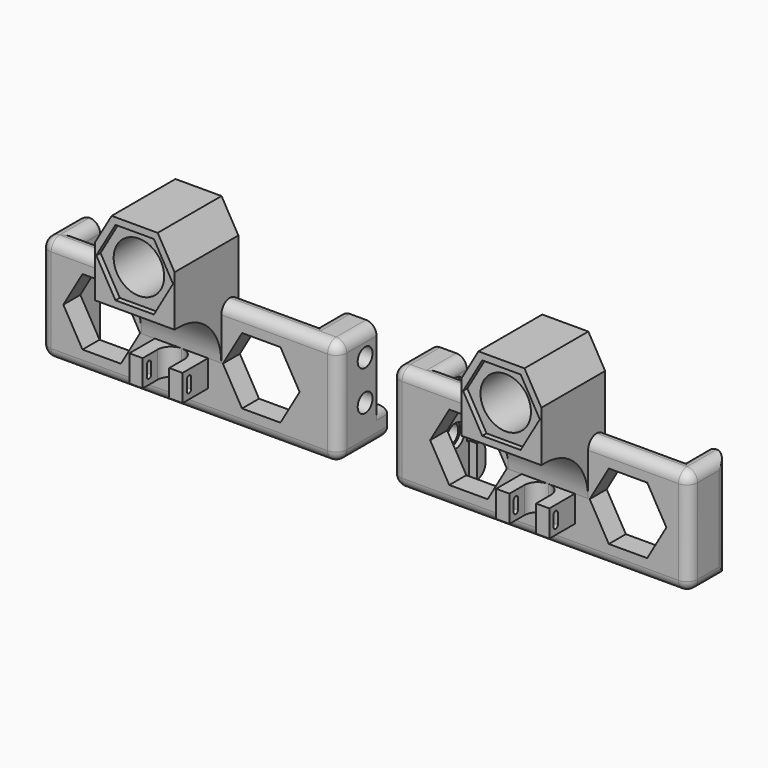
from build123d import *

# Parameters (mm, degrees)
F0_W          = 106
F0_H          = 40
F1_DEPTH      = 8
F2_W          = 8
F2_H          = 40
F2_W_2        = 5.97
F3_DEPTH      = 10
F3_DEPTH_BACK = 8
F4_W          = 13.97
F4_H          = 12
F5_DEPTH      = 5
F6_W          = 4
F6_H          = 12
F7_DEPTH      = 3
F8_W          = 30
F8_H          = 8
F9_DEPTH      = 30
F10_W         = 30
F10_H         = 30
F11_DEPTH     = 30
F12_R         = 9.5
F13_DEPTH     = 45.001
F15_DEPTH     = 2
F17_DEPTH     = 30.001
F19_DEPTH     = 2
F20_R         = 20
F21_R         = 3.99999
F24_DEPTH     = 10
F25_W         = 2
F25_H         = 4
F26_DEPTH     = 68.971
F27_R         = 3.4925
F28_DEPTH     = 13.2334
F29_R         = 4.318
F30_DEPTH     = 1.75
F32_DEPTH     = 23.001


# Not quite as in the source:
# - a fillet or chamfer is up to 0.001 mm smaller than in the source, because OpenCascade refuses the exact size


with BuildPart() as f1:
    # F0 (on Front) → F1 (new body)
    with BuildSketch(Plane.XZ):
        Rectangle(F0_W, F0_H)
    extrude(amount=F1_DEPTH)

    # F2 (on face) → F3 (join, two sides)
    with BuildSketch(Plane(origin=(0, 0, 0), x_dir=(-1, 0, 0), z_dir=(0, 1, 0))) as f3_sk:
        with Locations((-49, 0)):
            Rectangle(F2_W, F2_H)
        with Locations((-55.985, 0)):
            Rectangle(F2_W_2, F2_H)
        with Locations((49, 0)):
            Rectangle(F2_W, F2_H)
    extrude(amount=F3_DEPTH)
    extrude(f3_sk.sketch, amount=-F3_DEPTH_BACK)

    # F4 (on face) → F5 (join)
    with BuildSketch(Plane(origin=(0, 10, 0), x_dir=(-1, 0, 0), z_dir=(0, 1, 0))):
        with Locations((-51.985, -14)):
            Rectangle(F4_W, F4_H)
    extrude(amount=F5_DEPTH)

    # F6 (on face) → F7 (join)
    with BuildSketch(Plane(origin=(45, 0, 0), x_dir=(0, -1, 0), z_dir=(-1, 0, 0))):
        with Locations((-13, -14)):
            Rectangle(F6_W, F6_H)
    extrude(amount=F7_DEPTH)

    # F8 (on face) → F9 (join)
    with BuildSketch(Plane.XY.offset(20)):
        with Locations((0, -4)):
            Rectangle(F8_W, F8_H)
    extrude(amount=F9_DEPTH)

    # F10 (on face) → F11 (join)
    with BuildSketch(Plane(origin=(0, 0, 0), x_dir=(-1, 0, 0), z_dir=(0, 1, 0))):
        with Locations((0, 35)):
            Rectangle(F10_W, F10_H)
    extrude(amount=-F11_DEPTH)

    # F12 (on face) → F13 (cut, through all)
    with BuildSketch(Plane.XZ.offset(30)):
        with Locations((0, 35)):
            Circle(F12_R)
    extrude(amount=-F13_DEPTH, mode=Mode.SUBTRACT)

    # F14 (on face) → F15 (cut)
    with BuildSketch(Plane(origin=(0, 0, 0), x_dir=(-1, 0, 0), z_dir=(0, 1, 0))):
        Polygon((7.2890471485, 47.625), (-7.2890471485, 47.625), (-14.578094297, 35), (-7.2890471485, 22.375), (7.2890471485, 22.375), (14.578094297, 35), align=None)
    extrude(amount=-F15_DEPTH, mode=Mode.SUBTRACT)

    # F16 (on face) → F17 (cut, through all)
    with BuildSketch(Plane(origin=(0, 0, 0), x_dir=(-1, 0, 0), z_dir=(0, 1, 0))):
        Polygon((-18.9960915595, 39.0192378865), (-15, 39.0192378865), (-8.6602540378, 50), (8.6602540378, 50), (15, 39.0192378865), (19.5513442159, 39.0192378865), (19.5513442159, 53.0982163356), (-18.9960915595, 53.0982163356), align=None)
    extrude(amount=-F17_DEPTH, mode=Mode.SUBTRACT)

    # F18 (on face) → F19 (cut)
    with BuildSketch(Plane.XZ.offset(30)):
        Polygon((7.2168783649, 47.5), (-7.2168783649, 47.5), (-14.4337567297, 35), (-7.2168783649, 22.5), (7.2168783649, 22.5), (14.4337567297, 35), align=None)
    extrude(amount=-F19_DEPTH, mode=Mode.SUBTRACT)

    # F20
    f20_edges = [f1.edges().sort_by_distance(p)[0] for p in [
        (0, -8, 20),
    ]]
    fillet(f20_edges, radius=F20_R)

    # F21 (radius 4 in the source; OpenCascade refuses exactly that, so slightly less here)
    f21_edges = [f1.edges().sort_by_distance(p)[0] for p in [
        (-34, -8, 20),
        (30, 0, 20),
        (-30, 0, 20),
        (-53, -8, 0),
        (58.97, -8, 0),
        (58.97, 12.5, -8),
        (50.485, 15, -8),
        (50.485, 15, -20),
        (58.97, 1, 20),
        (36.985, -8, 20),
        (-53, 10, 0),
        (-45, 5, 20),
        (-53, 1, 20),
        (45, 5, 20),
        (2.985, -8, -20),
        (-53, 1, -20),
        (58.97, 3.5, -20),
    ]]
    fillet(f21_edges, radius=F21_R)

    # F23 (on offset) → F24 (join)
    with BuildSketch(Plane(origin=(0, 0, 0), x_dir=(1, 0, 0), z_dir=(0, 0, -1))):
        with BuildLine():
            Line((-5, 20), (-10, 20))
            Line((-10, 20), (-10, 8))
            Line((-10, 8), (0, 8))
            ThreePointArc((0, 8), (-3.5355339059, 9.4644660941), (-5, 13))
            Line((-5, 13), (-5, 20))
        make_face()
        with BuildLine():
            ThreePointArc((5, 13), (3.5355339059, 9.4644660941), (0, 8))
            Line((0, 8), (10, 8))
            Line((10, 8), (10, 20))
            Line((10, 20), (5, 20))
            Line((5, 20), (5, 13))
        make_face()
    extrude(amount=F24_DEPTH)

    # F25 (on face) → F26 (cut, through all)
    with BuildSketch(Plane(origin=(-10, 0, 0), x_dir=(0, -1, 0), z_dir=(-1, 0, 0))):
        with Locations((17, -5)):
            Rectangle(F25_W, F25_H)
        with BuildLine():
            Line((16, -3), (18, -3))
            ThreePointArc((18, -3), (17, -2), (16, -3))
        make_face()
        with BuildLine():
            ThreePointArc((16, -7), (17, -8), (18, -7))
            Line((18, -7), (16, -7))
        make_face()
    extrude(amount=-F26_DEPTH, mode=Mode.SUBTRACT)

    # F27 (on face) → F28 (cut)
    with BuildSketch(Plane.YZ.offset(58.97)):
        with Locations((4.6241632663, 11.0550189205)):
            Circle(F27_R)
        with Locations((4.6241632663, -3.9449810795)):
            Circle(F27_R)
    extrude(amount=-F28_DEPTH, mode=Mode.SUBTRACT)

    # F29 (on face) → F30 (cut)
    with BuildSketch(Plane(origin=(45, 0, 0), x_dir=(0, -1, 0), z_dir=(-1, 0, 0))):
        with Locations((-4.6241632663, 11.0550189205)):
            Circle(F29_R)
        with Locations((-4.6241632663, -3.9449810795)):
            Circle(F29_R)
    extrude(amount=-F30_DEPTH, mode=Mode.SUBTRACT)

    # F31 (on face) → F32 (cut, through all)
    with BuildSketch(Plane.XZ.offset(8)):
        Polygon((-22.7831216351, 12.5), (-37.2168783649, 12.5), (-44.4337567297, 0), (-37.2168783649, -12.5), (-22.7831216351, -12.5), (-15.5662432703, 0), align=None)
        Polygon((37.2168783649, 12.5), (22.7831216351, 12.5), (15.5662432703, 0), (22.7831216351, -12.5), (37.2168783649, -12.5), (44.4337567297, 0), align=None)
    extrude(amount=-F32_DEPTH, mode=Mode.SUBTRACT)


with BuildPart() as f34_1:
    # F34: instance of F1
    add(f1.part.mirror(Plane(origin=(68.97, 3.167424978, -1.4116276816), x_dir=(0, 1, 0), z_dir=(1, 0, 0))))


solid = Compound([f1.part, f34_1.part])
